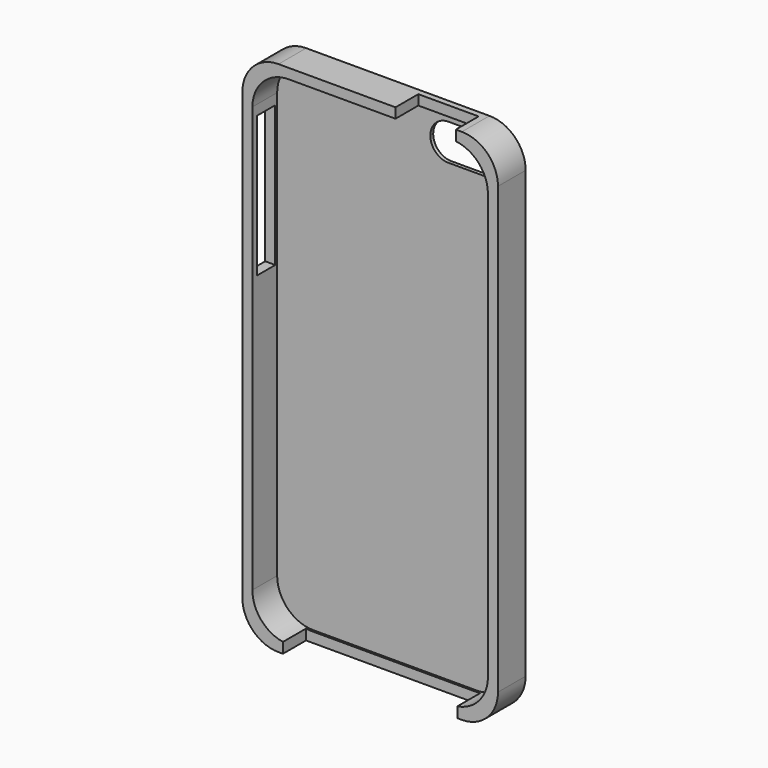
from build123d import *

# Parameters (mm, degrees)
F1_DEPTH  = 8.6
F3_DEPTH  = 7.7
F5_DEPTH  = 5
F7_DEPTH  = 1
F8_W      = 43.4
F8_H      = 7.1749998596
F9_DEPTH  = 25
F10_W     = 15
F10_H     = 7.1
F11_DEPTH = 25
F12_W     = 5.6
F12_H     = 35
F13_DEPTH = 25
F15_DEPTH = 1
F17_DEPTH = 0.95


# Not quite as in the source:
# - a feature names something its author has since deleted; it is built from what else it names


with BuildPart() as f1:
    # F0 (on Front) → F1 (new body)
    with BuildSketch(Plane.XZ):
        with BuildLine():
            Line((34.2577553943, 74.9795119995), (-11.3422446057, 74.9795119995))
            ThreePointArc((-11.3422446057, 74.9795119995), (-17.7062056364, 72.3434730302), (-20.3422446057, 65.9795119995))
            Line((-20.3422446057, 65.9795119995), (-20.3422446057, -44.8204880005))
            ThreePointArc((-20.3422446057, -44.8204880005), (-17.7062056364, -51.1844490312), (-11.3422446057, -53.8204880005))
            Line((-11.3422446057, -53.8204880005), (34.2577553943, -53.8204880005))
            ThreePointArc((34.2577553943, -53.8204880005), (40.621716425, -51.1844490312), (43.2577553943, -44.8204880005))
            Line((43.2577553943, -44.8204880005), (43.2577553943, 65.9795119995))
            ThreePointArc((43.2577553943, 65.9795119995), (40.621716425, 72.3434730302), (34.2577553943, 74.9795119995))
        make_face()
    extrude(amount=F1_DEPTH)

    # F2 (on face) → F3 (cut)
    with BuildSketch(Plane.XZ.offset(8.6)):
        with BuildLine():
            Line((31.7577553943, 72.4795119995), (-8.8422446057, 72.4795119995))
            ThreePointArc((-8.8422446057, 72.4795119995), (-15.2062056364, 69.8434730302), (-17.8422446057, 63.4795119995))
            Line((-17.8422446057, 63.4795119995), (-17.8422446057, -42.3204880005))
            ThreePointArc((-17.8422446057, -42.3204880005), (-15.2062056364, -48.6844490312), (-8.8422446057, -51.3204880005))
            Line((-8.8422446057, -51.3204880005), (31.7577553943, -51.3204880005))
            ThreePointArc((31.7577553943, -51.3204880005), (38.121716425, -48.6844490312), (40.7577553943, -42.3204880005))
            Line((40.7577553943, -42.3204880005), (40.7577553943, 63.4795119995))
            ThreePointArc((40.7577553943, 63.4795119995), (38.121716425, 69.8434730302), (31.7577553943, 72.4795119995))
        make_face()
    extrude(amount=-F3_DEPTH, mode=Mode.SUBTRACT)

    # F4 (on face) → F5 (cut)
    with BuildSketch(Plane(origin=(0, 0, 0), x_dir=(-1, 0, 0), z_dir=(0, 1, 0))):
        with BuildLine():
            Line((-24.7577553943, 70.9795119995), (-33.7577553943, 70.9795119995))
            ThreePointArc((-33.7577553943, 70.9795119995), (-36.9397359096, 69.6614925148), (-38.2577553943, 66.4795119995))
            ThreePointArc((-38.2577553943, 66.4795119995), (-36.9397359096, 63.2975314842), (-33.7577553943, 61.9795119995))
            Line((-33.7577553943, 61.9795119995), (-24.7577553943, 61.9795119995))
            ThreePointArc((-24.7577553943, 61.9795119995), (-21.5757748789, 63.2975314842), (-20.2577553943, 66.4795119995))
            ThreePointArc((-20.2577553943, 66.4795119995), (-21.5757748789, 69.6614925148), (-24.7577553943, 70.9795119995))
        make_face()
    extrude(amount=-F5_DEPTH, mode=Mode.SUBTRACT)

    # F6 (on face) → F7 (join)
    with BuildSketch(Plane(origin=(0, 0, 0), x_dir=(-1, 0, 0), z_dir=(0, 1, 0))):
        Polygon((-24.8744231037, 36.9551813005), (-26.7878402656, 32.3357836379), (-13.3939201328, 0), (0, 32.3357836379), (-1.9134171618, 36.9551813005), align=None)
    extrude(amount=F7_DEPTH)

    # F8 (on face) → F9 (cut)
    with BuildSketch(Plane(origin=(0, 0, -53.8204880005), x_dir=(1, 0, 0), z_dir=(0, 0, -1))):
        with Locations((11.4577553943, 5.0125000702)):
            Rectangle(F8_W, F8_H)
    extrude(amount=-F9_DEPTH, mode=Mode.SUBTRACT)

    # F10 (on face) → F11 (cut)
    with BuildSketch(Plane.XY.offset(74.9795119995)):
        with Locations((25.2577553943, -5.05)):
            Rectangle(F10_W, F10_H)
    extrude(amount=-F11_DEPTH, mode=Mode.SUBTRACT)

    # F12 (on face) → F13 (cut)
    with BuildSketch(Plane(origin=(-20.3422446057, 0, 0), x_dir=(0, -1, 0), z_dir=(-1, 0, 0))):
        with Locations((4.3, 43.4795119995)):
            Rectangle(F12_W, F12_H)
    extrude(amount=-F13_DEPTH, mode=Mode.SUBTRACT)

    # F14 (on face) → F15 (join)
    with BuildSketch(Plane(origin=(0, 1, 0), x_dir=(-1, 0, 0), z_dir=(0, 1, 0))):
        Polygon((-24.8744231037, 36.9551813005), (-26.7878402656, 32.3357836379), (0, 32.3357836379), (-1.9134171618, 36.9551813005), align=None)
    extrude(amount=F15_DEPTH)

    # F16 (on face) → F17 (join)
    with BuildSketch(Plane(origin=(0, 1, 0), x_dir=(-1, 0, 0), z_dir=(0, 1, 0))):
        Polygon((0, 32.3357836379), (-26.7878402656, 32.3357836379), (-13.3939201328, 0), align=None)
    extrude(amount=F17_DEPTH)


solid = f1.part
